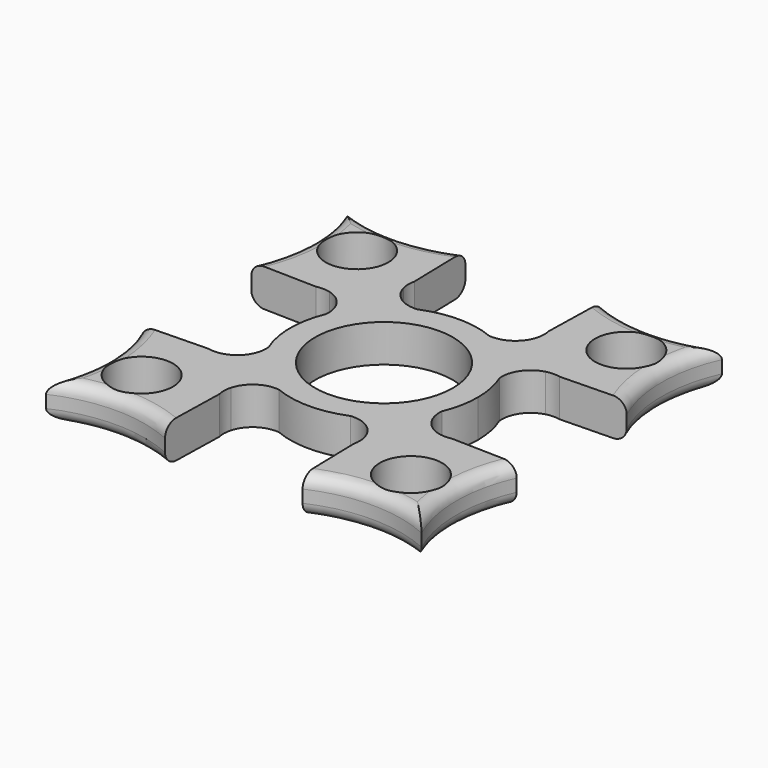
from build123d import *

# Parameters (mm, degrees)
F0_R         = 5
F0_R_2       = 11
F1_DEPTH     = 6
F2_T2_ANGLE  = 73.2799075376
F2_T4_ANGLE  = 73.2799075376
F2_T6_ANGLE  = 73.2799075376
F2_T8_ANGLE  = 73.2799075376
F2_T10_ANGLE = 73.2799075376
F2_T12_ANGLE = 73.2799075376
F2_T14_ANGLE = 73.2799075376
F2_T16_ANGLE = 73.2799075376
F2_T18_ANGLE = 73.2799075376
F2_T20_ANGLE = 73.2799075376
F2_T22_ANGLE = 73.2799075376
F2_T24_ANGLE = 73.2799075376
F2_T26_ANGLE = 73.2799075376
F2_T28_ANGLE = 73.2799075376
F2_T30_ANGLE = 73.2799075376
F2_T32_ANGLE = 73.2799075376


# Not quite as in the source:
# - a fillet or chamfer that OpenCascade refuses, or shapes differently, is made with other operations: its cross-section is extruded or revolved along the edge and cut away or added
# - a feature names something its author has since deleted; it is built from what else it names


with BuildPart() as f1:
    # F0 (on Top) → F1 (new body)
    with BuildSketch(Plane.XY):
        with BuildLine():
            ThreePointArc((10.9876487404, -30), (20.4938243702, -27.9570653866), (30, -30))
            ThreePointArc((30, -30), (27.9570653866, -20.4938243702), (30, -10.9876487404))
            Line((30, -10.9876487404), (19.4804511326, -10.7383985774))
            Line((19.4804511326, -10.7383985774), (12.3571271966, -12.3571271966))
            Line((12.3571271966, -12.3571271966), (10.7383985774, -19.4804511326))
            Line((10.7383985774, -19.4804511326), (10.9876487404, -30))
        make_face()
        with Locations((21.5147186258, -21.5147186258)):
            Circle(F0_R, mode=Mode.SUBTRACT)
        with BuildLine():
            ThreePointArc((-30, -30), (-20.4938243702, -27.9570653866), (-10.9876487404, -30))
            Line((-10.9876487404, -30), (-10.7383985774, -19.4804511326))
            Line((-10.7383985774, -19.4804511326), (-12.3571271966, -12.3571271966))
            Line((-12.3571271966, -12.3571271966), (-19.4804511326, -10.7383985774))
            Line((-19.4804511326, -10.7383985774), (-30, -10.9876487404))
            ThreePointArc((-30, -10.9876487404), (-27.9570653866, -20.4938243702), (-30, -30))
        make_face()
        with Locations((-21.5147186258, -21.5147186258)):
            Circle(F0_R, mode=Mode.SUBTRACT)
        with BuildLine():
            ThreePointArc((10.6848503434, -17.2204595732), (10.8519721537, -18.347129955), (10.7383985774, -19.4804511326))
            Line((10.7383985774, -19.4804511326), (12.3571271966, -12.3571271966))
            Line((12.3571271966, -12.3571271966), (10.5791915076, -12.7611514146))
            Line((10.5791915076, -12.7611514146), (10.6848503434, -17.2204595732))
        make_face()
        with BuildLine():
            Line((19.4804511326, 10.7383985774), (30, 10.9876487404))
            ThreePointArc((30, 10.9876487404), (27.9570653866, 20.4938243702), (30, 30))
            ThreePointArc((30, 30), (20.4938243702, 27.9570653866), (10.9876487404, 30))
            Line((10.9876487404, 30), (10.7383985774, 19.4804511326))
            Line((10.7383985774, 19.4804511326), (12.3571271966, 12.3571271966))
            Line((12.3571271966, 12.3571271966), (19.4804511326, 10.7383985774))
        make_face()
        with Locations((21.5147186258, 21.5147186258)):
            Circle(F0_R, mode=Mode.SUBTRACT)
        with BuildLine():
            Line((12.3571271966, -12.3571271966), (19.4804511326, -10.7383985774))
            ThreePointArc((19.4804511326, -10.7383985774), (18.347129955, -10.8519721537), (17.2204595732, -10.6848503434))
            Line((17.2204595732, -10.6848503434), (12.7611514146, -10.5791915076))
            Line((12.7611514146, -10.5791915076), (12.3571271966, -12.3571271966))
        make_face()
        with BuildLine():
            Line((-12.3571271966, -12.3571271966), (-10.7383985774, -19.4804511326))
            ThreePointArc((-10.7383985774, -19.4804511326), (-10.8519721537, -18.347129955), (-10.6848503434, -17.2204595732))
            Line((-10.6848503434, -17.2204595732), (-10.5791915076, -12.7611514146))
            Line((-10.5791915076, -12.7611514146), (-12.3571271966, -12.3571271966))
        make_face()
        with BuildLine():
            ThreePointArc((5.7264318341, -13.8639092052), (8.8229111996, -14.6303304894), (10.6848503434, -17.2204595732))
            Line((10.6848503434, -17.2204595732), (10.5791915076, -12.7611514146))
            Line((10.5791915076, -12.7611514146), (5.7264318341, -13.8639092052))
        make_face()
        with BuildLine():
            Line((10.5791915076, -12.7611514146), (12.3571271966, -12.3571271966))
            Line((12.3571271966, -12.3571271966), (12.7611514146, -10.5791915076))
            Line((12.7611514146, -10.5791915076), (10.6827084902, -10.5299448865))
            ThreePointArc((10.6827084902, -10.5299448865), (10.6066017178, -10.6066017178), (10.5299448865, -10.6827084902))
            Line((10.5299448865, -10.6827084902), (10.5791915076, -12.7611514146))
        make_face()
        with BuildLine():
            ThreePointArc((17.2204595732, 10.6848503434), (18.347129955, 10.8519721537), (19.4804511326, 10.7383985774))
            Line((19.4804511326, 10.7383985774), (12.3571271966, 12.3571271966))
            Line((12.3571271966, 12.3571271966), (12.7611514146, 10.5791915076))
            Line((12.7611514146, 10.5791915076), (17.2204595732, 10.6848503434))
        make_face()
        with BuildLine():
            Line((12.7611514146, -10.5791915076), (17.2204595732, -10.6848503434))
            ThreePointArc((17.2204595732, -10.6848503434), (14.6303304894, -8.8229111996), (13.8639092052, -5.7264318341))
            Line((13.8639092052, -5.7264318341), (12.7611514146, -10.5791915076))
        make_face()
        with BuildLine():
            Line((-10.5791915076, -12.7611514146), (-10.6848503434, -17.2204595732))
            ThreePointArc((-10.6848503434, -17.2204595732), (-8.8229111996, -14.6303304894), (-5.7264318341, -13.8639092052))
            Line((-5.7264318341, -13.8639092052), (-10.5791915076, -12.7611514146))
        make_face()
        with BuildLine():
            Line((-12.7611514146, -10.5791915076), (-12.3571271966, -12.3571271966))
            Line((-12.3571271966, -12.3571271966), (-10.5791915076, -12.7611514146))
            Line((-10.5791915076, -12.7611514146), (-10.5299448865, -10.6827084902))
            ThreePointArc((-10.5299448865, -10.6827084902), (-10.6066017178, -10.6066017178), (-10.6827084902, -10.5299448865))
            Line((-10.6827084902, -10.5299448865), (-12.7611514146, -10.5791915076))
        make_face()
        with BuildLine():
            Line((-19.4804511326, -10.7383985774), (-12.3571271966, -12.3571271966))
            Line((-12.3571271966, -12.3571271966), (-12.7611514146, -10.5791915076))
            Line((-12.7611514146, -10.5791915076), (-17.2204595732, -10.6848503434))
            ThreePointArc((-17.2204595732, -10.6848503434), (-18.347129955, -10.8519721537), (-19.4804511326, -10.7383985774))
        make_face()
        with BuildLine():
            Line((5.7264318341, -13.8639092052), (10.5791915076, -12.7611514146))
            Line((10.5791915076, -12.7611514146), (10.5299448865, -10.6827084902))
            ThreePointArc((10.5299448865, -10.6827084902), (8.2823580892, -12.5061002908), (5.7264318341, -13.8639092052))
        make_face()
        with BuildLine():
            ThreePointArc((-5.7264318341, -13.8639092052), (0, -15), (5.7264318341, -13.8639092052))
            ThreePointArc((5.7264318341, -13.8639092052), (8.2823580892, -12.5061002908), (10.5299448865, -10.6827084902))
            ThreePointArc((10.5299448865, -10.6827084902), (10.6066017178, -10.6066017178), (10.6827084902, -10.5299448865))
            ThreePointArc((10.6827084902, -10.5299448865), (12.5061002908, -8.2823580892), (13.8639092052, -5.7264318341))
            ThreePointArc((13.8639092052, -5.7264318341), (14.7132361851, -2.9190205483), (15, 0))
            ThreePointArc((15, 0), (14.7132361851, 2.9190205483), (13.8639092052, 5.7264318341))
            ThreePointArc((13.8639092052, 5.7264318341), (12.5061002908, 8.2823580892), (10.6827084902, 10.5299448865))
            ThreePointArc((10.6827084902, 10.5299448865), (10.6066017178, 10.6066017178), (10.5299448865, 10.6827084902))
            ThreePointArc((10.5299448865, 10.6827084902), (8.2823580892, 12.5061002908), (5.7264318341, 13.8639092052))
            ThreePointArc((5.7264318341, 13.8639092052), (0, 15), (-5.7264318341, 13.8639092052))
            ThreePointArc((-5.7264318341, 13.8639092052), (-8.2823580892, 12.5061002908), (-10.5299448865, 10.6827084902))
            ThreePointArc((-10.5299448865, 10.6827084902), (-10.6066017178, 10.6066017178), (-10.6827084902, 10.5299448865))
            ThreePointArc((-10.6827084902, 10.5299448865), (-12.5061002908, 8.2823580892), (-13.8639092052, 5.7264318341))
            ThreePointArc((-13.8639092052, 5.7264318341), (-15, 0), (-13.8639092052, -5.7264318341))
            ThreePointArc((-13.8639092052, -5.7264318341), (-12.5061002908, -8.2823580892), (-10.6827084902, -10.5299448865))
            ThreePointArc((-10.6827084902, -10.5299448865), (-10.6066017178, -10.6066017178), (-10.5299448865, -10.6827084902))
            ThreePointArc((-10.5299448865, -10.6827084902), (-8.2823580892, -12.5061002908), (-5.7264318341, -13.8639092052))
        make_face()
        Circle(F0_R_2, mode=Mode.SUBTRACT)
        with BuildLine():
            Line((10.6827084902, -10.5299448865), (12.7611514146, -10.5791915076))
            Line((12.7611514146, -10.5791915076), (13.8639092052, -5.7264318341))
            ThreePointArc((13.8639092052, -5.7264318341), (12.5061002908, -8.2823580892), (10.6827084902, -10.5299448865))
        make_face()
        with BuildLine():
            ThreePointArc((13.8639092052, 5.7264318341), (14.6303304894, 8.8229111996), (17.2204595732, 10.6848503434))
            Line((17.2204595732, 10.6848503434), (12.7611514146, 10.5791915076))
            Line((12.7611514146, 10.5791915076), (13.8639092052, 5.7264318341))
        make_face()
        with BuildLine():
            Line((10.5791915076, 12.7611514146), (12.3571271966, 12.3571271966))
            Line((12.3571271966, 12.3571271966), (10.7383985774, 19.4804511326))
            ThreePointArc((10.7383985774, 19.4804511326), (10.8519721537, 18.347129955), (10.6848503434, 17.2204595732))
            Line((10.6848503434, 17.2204595732), (10.5791915076, 12.7611514146))
        make_face()
        with BuildLine():
            Line((12.7611514146, 10.5791915076), (12.3571271966, 12.3571271966))
            Line((12.3571271966, 12.3571271966), (10.5791915076, 12.7611514146))
            Line((10.5791915076, 12.7611514146), (10.5299448865, 10.6827084902))
            ThreePointArc((10.5299448865, 10.6827084902), (10.6066017178, 10.6066017178), (10.6827084902, 10.5299448865))
            Line((10.6827084902, 10.5299448865), (12.7611514146, 10.5791915076))
        make_face()
        with BuildLine():
            ThreePointArc((-30, 30), (-27.9570653866, 20.4938243702), (-30, 10.9876487404))
            Line((-30, 10.9876487404), (-19.4804511326, 10.7383985774))
            Line((-19.4804511326, 10.7383985774), (-12.3571271966, 12.3571271966))
            Line((-12.3571271966, 12.3571271966), (-10.7383985774, 19.4804511326))
            Line((-10.7383985774, 19.4804511326), (-10.9876487404, 30))
            ThreePointArc((-10.9876487404, 30), (-20.4938243702, 27.9570653866), (-30, 30))
        make_face()
        with Locations((-21.5147186258, 21.5147186258)):
            Circle(F0_R, mode=Mode.SUBTRACT)
        with BuildLine():
            Line((-10.5299448865, -10.6827084902), (-10.5791915076, -12.7611514146))
            Line((-10.5791915076, -12.7611514146), (-5.7264318341, -13.8639092052))
            ThreePointArc((-5.7264318341, -13.8639092052), (-8.2823580892, -12.5061002908), (-10.5299448865, -10.6827084902))
        make_face()
        with BuildLine():
            Line((-13.8639092052, -5.7264318341), (-12.7611514146, -10.5791915076))
            Line((-12.7611514146, -10.5791915076), (-10.6827084902, -10.5299448865))
            ThreePointArc((-10.6827084902, -10.5299448865), (-12.5061002908, -8.2823580892), (-13.8639092052, -5.7264318341))
        make_face()
        with BuildLine():
            Line((-17.2204595732, -10.6848503434), (-12.7611514146, -10.5791915076))
            Line((-12.7611514146, -10.5791915076), (-13.8639092052, -5.7264318341))
            ThreePointArc((-13.8639092052, -5.7264318341), (-14.6303304894, -8.8229111996), (-17.2204595732, -10.6848503434))
        make_face()
        with BuildLine():
            Line((13.8639092052, 5.7264318341), (12.7611514146, 10.5791915076))
            Line((12.7611514146, 10.5791915076), (10.6827084902, 10.5299448865))
            ThreePointArc((10.6827084902, 10.5299448865), (12.5061002908, 8.2823580892), (13.8639092052, 5.7264318341))
        make_face()
        with BuildLine():
            Line((5.7264318341, 13.8639092052), (10.5791915076, 12.7611514146))
            Line((10.5791915076, 12.7611514146), (10.6848503434, 17.2204595732))
            ThreePointArc((10.6848503434, 17.2204595732), (8.8229111996, 14.6303304894), (5.7264318341, 13.8639092052))
        make_face()
        with BuildLine():
            Line((10.5299448865, 10.6827084902), (10.5791915076, 12.7611514146))
            Line((10.5791915076, 12.7611514146), (5.7264318341, 13.8639092052))
            ThreePointArc((5.7264318341, 13.8639092052), (8.2823580892, 12.5061002908), (10.5299448865, 10.6827084902))
        make_face()
        with BuildLine():
            Line((-12.3571271966, 12.3571271966), (-19.4804511326, 10.7383985774))
            ThreePointArc((-19.4804511326, 10.7383985774), (-18.347129955, 10.8519721537), (-17.2204595732, 10.6848503434))
            Line((-17.2204595732, 10.6848503434), (-12.7611514146, 10.5791915076))
            Line((-12.7611514146, 10.5791915076), (-12.3571271966, 12.3571271966))
        make_face()
        with BuildLine():
            ThreePointArc((-10.6848503434, 17.2204595732), (-10.8519721537, 18.347129955), (-10.7383985774, 19.4804511326))
            Line((-10.7383985774, 19.4804511326), (-12.3571271966, 12.3571271966))
            Line((-12.3571271966, 12.3571271966), (-10.5791915076, 12.7611514146))
            Line((-10.5791915076, 12.7611514146), (-10.6848503434, 17.2204595732))
        make_face()
        with BuildLine():
            Line((-12.7611514146, 10.5791915076), (-17.2204595732, 10.6848503434))
            ThreePointArc((-17.2204595732, 10.6848503434), (-14.6303304894, 8.8229111996), (-13.8639092052, 5.7264318341))
            Line((-13.8639092052, 5.7264318341), (-12.7611514146, 10.5791915076))
        make_face()
        with BuildLine():
            Line((-10.5791915076, 12.7611514146), (-12.3571271966, 12.3571271966))
            Line((-12.3571271966, 12.3571271966), (-12.7611514146, 10.5791915076))
            Line((-12.7611514146, 10.5791915076), (-10.6827084902, 10.5299448865))
            ThreePointArc((-10.6827084902, 10.5299448865), (-10.6066017178, 10.6066017178), (-10.5299448865, 10.6827084902))
            Line((-10.5299448865, 10.6827084902), (-10.5791915076, 12.7611514146))
        make_face()
        with BuildLine():
            Line((-12.7611514146, 10.5791915076), (-13.8639092052, 5.7264318341))
            ThreePointArc((-13.8639092052, 5.7264318341), (-12.5061002908, 8.2823580892), (-10.6827084902, 10.5299448865))
            Line((-10.6827084902, 10.5299448865), (-12.7611514146, 10.5791915076))
        make_face()
        with BuildLine():
            ThreePointArc((-5.7264318341, 13.8639092052), (-8.8229111996, 14.6303304894), (-10.6848503434, 17.2204595732))
            Line((-10.6848503434, 17.2204595732), (-10.5791915076, 12.7611514146))
            Line((-10.5791915076, 12.7611514146), (-5.7264318341, 13.8639092052))
        make_face()
        with BuildLine():
            ThreePointArc((-10.5299448865, 10.6827084902), (-8.2823580892, 12.5061002908), (-5.7264318341, 13.8639092052))
            Line((-5.7264318341, 13.8639092052), (-10.5791915076, 12.7611514146))
            Line((-10.5791915076, 12.7611514146), (-10.5299448865, 10.6827084902))
        make_face()
    extrude(amount=F1_DEPTH)

    # F2: fillet of radius 2 on 16 edges, made by hand

    # F2_s1 → F2_t2 (revolve, cut)
    with BuildSketch(Plane(origin=(11.2727615438, 8.3840942821, 0), x_dir=(0, 0, 1), z_dir=(0.8024015176, 0.5967845545, 0))):
        with BuildLine():
            ThreePointArc((4, -30.0910535835), (5.4142135624, -29.5052671459), (6, -28.0910535835))
            Line((6, -28.0910535835), (6, -30.0910535835))
            Line((6, -30.0910535835), (4, -30.0910535835))
        make_face()
    revolve(axis=Axis((-20.4938243702, 51.0955829676, 6), (0, 0, -1)), revolution_arc=F2_T2_ANGLE, mode=Mode.SUBTRACT)

    # F2_s3 → F2_t4 (revolve, cut)
    with BuildSketch(Plane(origin=(-28.0114738694, 37.6625852232, 0), x_dir=(0, 0, 1), z_dir=(-0.5967845545, 0.8024015176, 0))):
        with BuildLine():
            ThreePointArc((4, -5.6302578897), (5.4142135624, -5.0444714521), (6, -3.6302578897))
            Line((6, -3.6302578897), (6, -5.6302578897))
            Line((6, -5.6302578897), (4, -5.6302578897))
        make_face()
    revolve(axis=Axis((-51.0955829676, 20.4938243702, 6), (0, 0, -1)), revolution_arc=F2_T4_ANGLE, mode=Mode.SUBTRACT)

    # F2_s5 → F2_t6 (revolve, cut)
    with BuildSketch(Plane(origin=(11.2727615438, 8.3840942821, 0), x_dir=(0, 0, 1), z_dir=(0.8024015176, 0.5967845545, 0))):
        with BuildLine():
            ThreePointArc((2, -30.0910535835), (0.5857864376, -29.5052671459), (0, -28.0910535835))
            Line((0, -28.0910535835), (0, -30.0910535835))
            Line((0, -30.0910535835), (2, -30.0910535835))
        make_face()
    revolve(axis=Axis((-20.4938243702, 51.0955829676, 0), (0, 0, -1)), revolution_arc=F2_T6_ANGLE, mode=Mode.SUBTRACT)

    # F2_s7 → F2_t8 (revolve, cut)
    with BuildSketch(Plane(origin=(-28.0114738694, 37.6625852232, 0), x_dir=(0, 0, 1), z_dir=(-0.5967845545, 0.8024015176, 0))):
        with BuildLine():
            ThreePointArc((2, -5.6302578897), (0.5857864376, -5.0444714521), (0, -3.6302578897))
            Line((0, -3.6302578897), (0, -5.6302578897))
            Line((0, -5.6302578897), (2, -5.6302578897))
        make_face()
    revolve(axis=Axis((-51.0955829676, 20.4938243702, 0), (0, 0, -1)), revolution_arc=F2_T8_ANGLE, mode=Mode.SUBTRACT)

    # F2_s9 → F2_t10 (revolve, cut)
    with BuildSketch(Plane(origin=(37.6625852232, 28.0114738694, 0), x_dir=(0, 0, 1), z_dir=(0.8024015176, 0.5967845545, 0))):
        with BuildLine():
            ThreePointArc((4, -5.6302578897), (5.4142135624, -5.0444714521), (6, -3.6302578897))
            Line((6, -3.6302578897), (6, -5.6302578897))
            Line((6, -5.6302578897), (4, -5.6302578897))
        make_face()
    revolve(axis=Axis((20.4938243702, 51.0955829676, 6), (0, 0, -1)), revolution_arc=F2_T10_ANGLE, mode=Mode.SUBTRACT)

    # F2_s11 → F2_t12 (revolve, cut)
    with BuildSketch(Plane(origin=(37.6625852232, 28.0114738694, 0), x_dir=(0, 0, 1), z_dir=(0.8024015176, 0.5967845545, 0))):
        with BuildLine():
            ThreePointArc((2, -5.6302578897), (0.5857864376, -5.0444714521), (0, -3.6302578897))
            Line((0, -3.6302578897), (0, -5.6302578897))
            Line((0, -5.6302578897), (2, -5.6302578897))
        make_face()
    revolve(axis=Axis((20.4938243702, 51.0955829676, 0), (0, 0, -1)), revolution_arc=F2_T12_ANGLE, mode=Mode.SUBTRACT)

    # F2_s13 → F2_t14 (revolve, cut)
    with BuildSketch(Plane(origin=(8.3840942821, -11.2727615438, 0), x_dir=(0, 0, 1), z_dir=(0.5967845545, -0.8024015176, 0))):
        with BuildLine():
            ThreePointArc((4, -30.0910535835), (5.4142135624, -29.5052671459), (6, -28.0910535835))
            Line((6, -28.0910535835), (6, -30.0910535835))
            Line((6, -30.0910535835), (4, -30.0910535835))
        make_face()
    revolve(axis=Axis((51.0955829676, 20.4938243702, 6), (0, 0, -1)), revolution_arc=F2_T14_ANGLE, mode=Mode.SUBTRACT)

    # F2_s15 → F2_t16 (revolve, cut)
    with BuildSketch(Plane(origin=(-8.3840942821, 11.2727615438, 0), x_dir=(0, 0, 1), z_dir=(-0.5967845545, 0.8024015176, 0))):
        with BuildLine():
            ThreePointArc((4, -30.0910535835), (5.4142135624, -29.5052671459), (6, -28.0910535835))
            Line((6, -28.0910535835), (6, -30.0910535835))
            Line((6, -30.0910535835), (4, -30.0910535835))
        make_face()
    revolve(axis=Axis((-51.0955829676, -20.4938243702, 6), (0, 0, -1)), revolution_arc=F2_T16_ANGLE, mode=Mode.SUBTRACT)

    # F2_s17 → F2_t18 (revolve, cut)
    with BuildSketch(Plane(origin=(28.0114738694, -37.6625852232, 0), x_dir=(0, 0, 1), z_dir=(0.5967845545, -0.8024015176, 0))):
        with BuildLine():
            ThreePointArc((4, -5.6302578897), (5.4142135624, -5.0444714521), (6, -3.6302578897))
            Line((6, -3.6302578897), (6, -5.6302578897))
            Line((6, -5.6302578897), (4, -5.6302578897))
        make_face()
    revolve(axis=Axis((51.0955829676, -20.4938243702, 6), (0, 0, -1)), revolution_arc=F2_T18_ANGLE, mode=Mode.SUBTRACT)

    # F2_s19 → F2_t20 (revolve, cut)
    with BuildSketch(Plane(origin=(-11.2727615438, -8.3840942821, 0), x_dir=(0, 0, 1), z_dir=(-0.8024015176, -0.5967845545, 0))):
        with BuildLine():
            ThreePointArc((4, -30.0910535835), (5.4142135624, -29.5052671459), (6, -28.0910535835))
            Line((6, -28.0910535835), (6, -30.0910535835))
            Line((6, -30.0910535835), (4, -30.0910535835))
        make_face()
    revolve(axis=Axis((20.4938243702, -51.0955829676, 6), (0, 0, -1)), revolution_arc=F2_T20_ANGLE, mode=Mode.SUBTRACT)

    # F2_s21 → F2_t22 (revolve, cut)
    with BuildSketch(Plane(origin=(-37.6625852232, -28.0114738694, 0), x_dir=(0, 0, 1), z_dir=(-0.8024015176, -0.5967845545, 0))):
        with BuildLine():
            ThreePointArc((4, -5.6302578897), (5.4142135624, -5.0444714521), (6, -3.6302578897))
            Line((6, -3.6302578897), (6, -5.6302578897))
            Line((6, -5.6302578897), (4, -5.6302578897))
        make_face()
    revolve(axis=Axis((-20.4938243702, -51.0955829676, 6), (0, 0, -1)), revolution_arc=F2_T22_ANGLE, mode=Mode.SUBTRACT)

    # F2_s23 → F2_t24 (revolve, cut)
    with BuildSketch(Plane(origin=(28.0114738694, -37.6625852232, 0), x_dir=(0, 0, 1), z_dir=(0.5967845545, -0.8024015176, 0))):
        with BuildLine():
            ThreePointArc((2, -5.6302578897), (0.5857864376, -5.0444714521), (0, -3.6302578897))
            Line((0, -3.6302578897), (0, -5.6302578897))
            Line((0, -5.6302578897), (2, -5.6302578897))
        make_face()
    revolve(axis=Axis((51.0955829676, -20.4938243702, 0), (0, 0, -1)), revolution_arc=F2_T24_ANGLE, mode=Mode.SUBTRACT)

    # F2_s25 → F2_t26 (revolve, cut)
    with BuildSketch(Plane(origin=(8.3840942821, -11.2727615438, 0), x_dir=(0, 0, 1), z_dir=(0.5967845545, -0.8024015176, 0))):
        with BuildLine():
            ThreePointArc((2, -30.0910535835), (0.5857864376, -29.5052671459), (0, -28.0910535835))
            Line((0, -28.0910535835), (0, -30.0910535835))
            Line((0, -30.0910535835), (2, -30.0910535835))
        make_face()
    revolve(axis=Axis((51.0955829676, 20.4938243702, 0), (0, 0, -1)), revolution_arc=F2_T26_ANGLE, mode=Mode.SUBTRACT)

    # F2_s27 → F2_t28 (revolve, cut)
    with BuildSketch(Plane(origin=(-11.2727615438, -8.3840942821, 0), x_dir=(0, 0, 1), z_dir=(-0.8024015176, -0.5967845545, 0))):
        with BuildLine():
            ThreePointArc((2, -30.0910535835), (0.5857864376, -29.5052671459), (0, -28.0910535835))
            Line((0, -28.0910535835), (0, -30.0910535835))
            Line((0, -30.0910535835), (2, -30.0910535835))
        make_face()
    revolve(axis=Axis((20.4938243702, -51.0955829676, 0), (0, 0, -1)), revolution_arc=F2_T28_ANGLE, mode=Mode.SUBTRACT)

    # F2_s29 → F2_t30 (revolve, cut)
    with BuildSketch(Plane(origin=(-37.6625852232, -28.0114738694, 0), x_dir=(0, 0, 1), z_dir=(-0.8024015176, -0.5967845545, 0))):
        with BuildLine():
            ThreePointArc((2, -5.6302578897), (0.5857864376, -5.0444714521), (0, -3.6302578897))
            Line((0, -3.6302578897), (0, -5.6302578897))
            Line((0, -5.6302578897), (2, -5.6302578897))
        make_face()
    revolve(axis=Axis((-20.4938243702, -51.0955829676, 0), (0, 0, -1)), revolution_arc=F2_T30_ANGLE, mode=Mode.SUBTRACT)

    # F2_s31 → F2_t32 (revolve, cut)
    with BuildSketch(Plane(origin=(-8.3840942821, 11.2727615438, 0), x_dir=(0, 0, 1), z_dir=(-0.5967845545, 0.8024015176, 0))):
        with BuildLine():
            ThreePointArc((2, -30.0910535835), (0.5857864376, -29.5052671459), (0, -28.0910535835))
            Line((0, -28.0910535835), (0, -30.0910535835))
            Line((0, -30.0910535835), (2, -30.0910535835))
        make_face()
    revolve(axis=Axis((-51.0955829676, -20.4938243702, 0), (0, 0, -1)), revolution_arc=F2_T32_ANGLE, mode=Mode.SUBTRACT)


solid = f1.part
